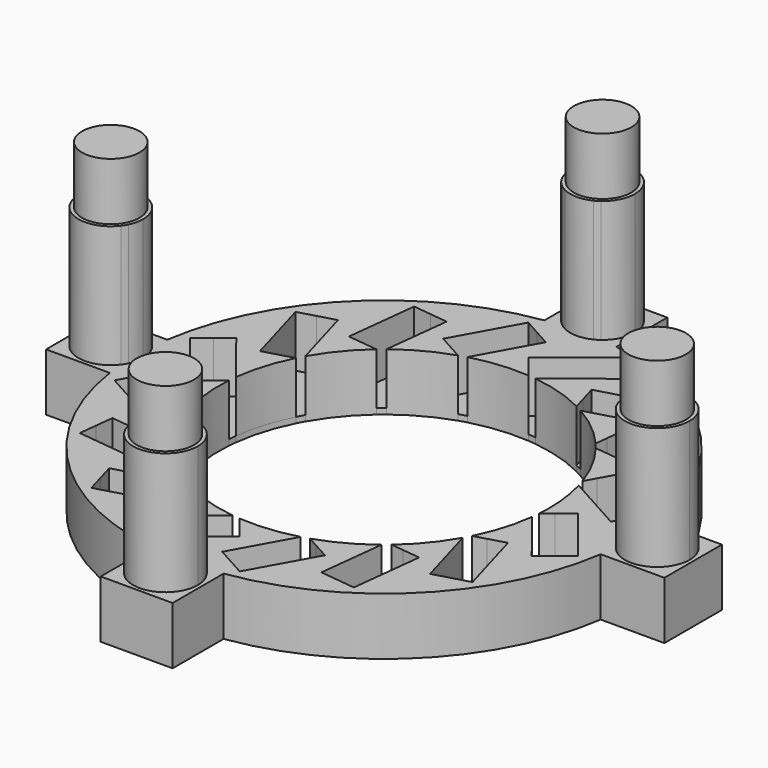
from build123d import *

# Parameters (mm, degrees)
F2_DEPTH = 8
F1_R     = 4
F3_DEPTH = 25
F4_DEPTH = 33
F5_DEPTH = 4
F0_R     = 34
F6_DEPTH = 0.8


# Not quite as in the source:
# - a feature names something its author has since deleted; it is built from what else it names


with BuildPart() as f2:
    # F1 (on Top) → F2 (new body)
    with BuildSketch(Plane.XY):
        with BuildLine():
            ThreePointArc((-33.944079, -1.949232), (-34.1514, -2.332012), (-34.394737, -2.692968))
            ThreePointArc((-34.394737, -2.692968), (-34.284658, -3.848663), (-34.135758, -5))
            ThreePointArc((-34.135758, -5), (-24.395184, -24.395184), (-5, -34.135758))
            ThreePointArc((-5, -34.135758), (-3.848663, -34.284658), (-2.692968, -34.394737))
            ThreePointArc((-2.692968, -34.394737), (-2.332012, -34.1514), (-1.949232, -33.944079))
            ThreePointArc((-1.949232, -33.944079), (-24.041631, -24.041631), (-33.944079, -1.949232))
        make_face()
        with BuildLine():
            ThreePointArc((-34.135758, -5), (-34.284658, -3.848663), (-34.394737, -2.692968))
            ThreePointArc((-34.394737, -2.692968), (-42.5, 0), (-34.394737, 2.692968))
            ThreePointArc((-34.394737, 2.692968), (-34.284658, 3.848663), (-34.135758, 5))
            Line((-34.135758, 5), (-43, 5))
            Line((-43, 5), (-43, 0))
            Line((-43, 0), (-43, -5))
            Line((-43, -5), (-34.135758, -5))
        make_face()
        with BuildLine():
            ThreePointArc((-34.135758, 5), (-34.284658, 3.848663), (-34.394737, 2.692968))
            ThreePointArc((-34.394737, 2.692968), (-34.1514, 2.332012), (-33.944079, 1.949232))
            ThreePointArc((-33.944079, 1.949232), (-24.041631, 24.041631), (-1.949232, 33.944079))
            ThreePointArc((-1.949232, 33.944079), (-2.332012, 34.1514), (-2.692968, 34.394737))
            ThreePointArc((-2.692968, 34.394737), (-3.848663, 34.284658), (-5, 34.135758))
            ThreePointArc((-5, 34.135758), (-24.395184, 24.395184), (-34.135758, 5))
        make_face()
        with BuildLine():
            ThreePointArc((-2.692968, -34.394737), (-3.848663, -34.284658), (-5, -34.135758))
            Line((-5, -34.135758), (-5, -43))
            Line((-5, -43), (0, -43))
            Line((0, -43), (5, -43))
            Line((5, -43), (5, -34.135758))
            ThreePointArc((5, -34.135758), (3.848663, -34.284658), (2.692968, -34.394737))
            ThreePointArc((2.692968, -34.394737), (4.022956, -35.983612), (4.5, -38))
            ThreePointArc((4.5, -38), (-2.016388, -42.022956), (-2.692968, -34.394737))
        make_face()
        with BuildLine():
            Line((-5, 43), (-5, 34.135758))
            ThreePointArc((-5, 34.135758), (-3.848663, 34.284658), (-2.692968, 34.394737))
            ThreePointArc((-2.692968, 34.394737), (-4.270462, 39.418858), (0, 42.5))
            Line((0, 42.5), (0, 43))
            Line((0, 43), (-5, 43))
        make_face()
        with BuildLine():
            ThreePointArc((33.944079, -1.949232), (24.041631, -24.041631), (1.949232, -33.944079))
            ThreePointArc((1.949232, -33.944079), (2.332012, -34.1514), (2.692968, -34.394737))
            ThreePointArc((2.692968, -34.394737), (3.848663, -34.284658), (5, -34.135758))
            ThreePointArc((5, -34.135758), (24.395184, -24.395184), (34.135758, -5))
            ThreePointArc((34.135758, -5), (34.284658, -3.848663), (34.394737, -2.692968))
            ThreePointArc((34.394737, -2.692968), (34.1514, -2.332012), (33.944079, -1.949232))
        make_face()
        with BuildLine():
            ThreePointArc((2.692968, 34.394737), (2.332012, 34.1514), (1.949232, 33.944079))
            ThreePointArc((1.949232, 33.944079), (24.041631, 24.041631), (33.944079, 1.949232))
            ThreePointArc((33.944079, 1.949232), (34.1514, 2.332012), (34.394737, 2.692968))
            ThreePointArc((34.394737, 2.692968), (34.284658, 3.848663), (34.135758, 5))
            ThreePointArc((34.135758, 5), (24.395184, 24.395184), (5, 34.135758))
            ThreePointArc((5, 34.135758), (3.848663, 34.284658), (2.692968, 34.394737))
        make_face()
        with BuildLine():
            Line((0, 43), (0, 42.5))
            ThreePointArc((0, 42.5), (3.181981, 41.181981), (4.5, 38))
            ThreePointArc((4.5, 38), (4.022956, 35.983612), (2.692968, 34.394737))
            ThreePointArc((2.692968, 34.394737), (3.848663, 34.284658), (5, 34.135758))
            Line((5, 34.135758), (5, 43))
            Line((5, 43), (0, 43))
        make_face()
        with BuildLine():
            ThreePointArc((42.5, 0), (39.418858, -4.270462), (34.394737, -2.692968))
            ThreePointArc((34.394737, -2.692968), (34.284658, -3.848663), (34.135758, -5))
            Line((34.135758, -5), (43, -5))
            Line((43, -5), (43, 0))
            Line((43, 0), (43, 5))
            Line((43, 5), (34.135758, 5))
            ThreePointArc((34.135758, 5), (34.284658, 3.848663), (34.394737, 2.692968))
            ThreePointArc((34.394737, 2.692968), (39.418858, 4.270462), (42.5, 0))
        make_face()
        with BuildLine():
            ThreePointArc((-33.5, 0), (-33.612424, -0.999589), (-33.944079, -1.949232))
            ThreePointArc((-33.944079, -1.949232), (-24.041631, -24.041631), (-1.949232, -33.944079))
            ThreePointArc((-1.949232, -33.944079), (0, -33.5), (1.949232, -33.944079))
            ThreePointArc((1.949232, -33.944079), (24.041631, -24.041631), (33.944079, -1.949232))
            ThreePointArc((33.944079, -1.949232), (33.5, 0), (33.944079, 1.949232))
            ThreePointArc((33.944079, 1.949232), (24.041631, 24.041631), (1.949232, 33.944079))
            ThreePointArc((1.949232, 33.944079), (0, 33.5), (-1.949232, 33.944079))
            ThreePointArc((-1.949232, 33.944079), (-24.041631, 24.041631), (-33.944079, 1.949232))
            ThreePointArc((-33.944079, 1.949232), (-33.612424, 0.999589), (-33.5, 0))
        make_face()
        with BuildLine():
            ThreePointArc((22.165631, 6.138794), (22.790453, 3.097618), (23, 0))
            ThreePointArc((23, 0), (22.98399, -0.858012), (22.935984, -1.71483))
            Line((22.935984, -1.71483), (24.292118, -0.636112))
            Line((24.292118, -0.636112), (26.248639, 0.920175))
            Line((26.248639, 0.920175), (32.473785, -6.905906))
            Line((32.473785, -6.905906), (30.517265, -8.462193))
            Line((30.517265, -8.462193), (28.560744, -10.01848))
            Line((28.560744, -10.01848), (22.827588, -2.810914))
            ThreePointArc((22.827588, -2.810914), (22.006964, -6.685323), (20.533849, -10.361517))
            Line((20.533849, -10.361517), (22.199562, -9.883882))
            Line((22.199562, -9.883882), (24.602716, -9.194788))
            Line((24.602716, -9.194788), (27.35909, -18.807405))
            Line((27.35909, -18.807405), (24.955935, -19.496499))
            Line((24.955935, -19.496499), (22.552781, -20.185592))
            Line((22.552781, -20.185592), (20.014251, -11.332685))
            ThreePointArc((20.014251, -11.332685), (17.773421, -14.598134), (15.005622, -17.430757))
            Line((15.005622, -17.430757), (16.727323, -17.62692))
            Line((16.727323, -17.62692), (19.211253, -17.909928))
            Line((19.211253, -17.909928), (18.07922, -27.845647))
            Line((18.07922, -27.845647), (15.595291, -27.562639))
            Line((15.595291, -27.562639), (13.111361, -27.279631))
            Line((13.111361, -27.279631), (14.153926, -18.129158))
            ThreePointArc((14.153926, -18.129158), (10.834036, -20.288511), (7.192925, -21.846323))
            Line((7.192925, -21.846323), (8.708501, -22.68642))
            Line((8.708501, -22.68642), (10.89505, -23.898444))
            Line((10.89505, -23.898444), (6.046954, -32.644642))
            Line((6.046954, -32.644642), (3.860405, -31.432617))
            Line((3.860405, -31.432617), (1.673855, -30.220593))
            Line((1.673855, -30.220593), (6.138794, -22.165631))
            ThreePointArc((6.138794, -22.165631), (2.245267, -22.890146), (-1.71483, -22.935984))
            Line((-1.71483, -22.935984), (-0.636112, -24.292118))
            Line((-0.636112, -24.292118), (0.920175, -26.248639))
            Line((0.920175, -26.248639), (-6.905906, -32.473785))
            Line((-6.905906, -32.473785), (-8.462193, -30.517265))
            Line((-8.462193, -30.517265), (-10.01848, -28.560744))
            Line((-10.01848, -28.560744), (-2.810914, -22.827588))
            ThreePointArc((-2.810914, -22.827588), (-6.685323, -22.006964), (-10.361517, -20.533849))
            Line((-10.361517, -20.533849), (-9.883882, -22.199562))
            Line((-9.883882, -22.199562), (-9.194788, -24.602716))
            Line((-9.194788, -24.602716), (-18.807405, -27.35909))
            Line((-18.807405, -27.35909), (-19.496499, -24.955935))
            Line((-19.496499, -24.955935), (-20.185592, -22.552781))
            Line((-20.185592, -22.552781), (-11.332685, -20.014251))
            ThreePointArc((-11.332685, -20.014251), (-14.598134, -17.773421), (-17.430757, -15.005622))
            Line((-17.430757, -15.005622), (-17.62692, -16.727323))
            Line((-17.62692, -16.727323), (-17.909928, -19.211253))
            Line((-17.909928, -19.211253), (-27.845647, -18.07922))
            Line((-27.845647, -18.07922), (-27.562639, -15.595291))
            Line((-27.562639, -15.595291), (-27.279631, -13.111361))
            Line((-27.279631, -13.111361), (-18.129158, -14.153926))
            ThreePointArc((-18.129158, -14.153926), (-20.288511, -10.834036), (-21.846323, -7.192925))
            Line((-21.846323, -7.192925), (-22.68642, -8.708501))
            Line((-22.68642, -8.708501), (-23.898444, -10.89505))
            Line((-23.898444, -10.89505), (-32.644642, -6.046954))
            Line((-32.644642, -6.046954), (-31.432617, -3.860405))
            Line((-31.432617, -3.860405), (-30.220593, -1.673855))
            Line((-30.220593, -1.673855), (-22.165631, -6.138794))
            ThreePointArc((-22.165631, -6.138794), (-22.890146, -2.245267), (-22.935984, 1.71483))
            Line((-22.935984, 1.71483), (-24.292118, 0.636112))
            Line((-24.292118, 0.636112), (-26.248639, -0.920175))
            Line((-26.248639, -0.920175), (-32.473785, 6.905906))
            Line((-32.473785, 6.905906), (-30.517265, 8.462193))
            Line((-30.517265, 8.462193), (-28.560744, 10.01848))
            Line((-28.560744, 10.01848), (-22.827588, 2.810914))
            ThreePointArc((-22.827588, 2.810914), (-22.006964, 6.685323), (-20.533849, 10.361517))
            Line((-20.533849, 10.361517), (-22.199562, 9.883882))
            Line((-22.199562, 9.883882), (-24.602716, 9.194788))
            Line((-24.602716, 9.194788), (-27.35909, 18.807405))
            Line((-27.35909, 18.807405), (-24.955935, 19.496499))
            Line((-24.955935, 19.496499), (-22.552781, 20.185592))
            Line((-22.552781, 20.185592), (-20.014251, 11.332685))
            ThreePointArc((-20.014251, 11.332685), (-17.773421, 14.598134), (-15.005622, 17.430757))
            Line((-15.005622, 17.430757), (-16.727323, 17.62692))
            Line((-16.727323, 17.62692), (-19.211253, 17.909928))
            Line((-19.211253, 17.909928), (-18.07922, 27.845647))
            Line((-18.07922, 27.845647), (-15.595291, 27.562639))
            Line((-15.595291, 27.562639), (-13.111361, 27.279631))
            Line((-13.111361, 27.279631), (-14.153926, 18.129158))
            ThreePointArc((-14.153926, 18.129158), (-10.834036, 20.288511), (-7.192925, 21.846323))
            Line((-7.192925, 21.846323), (-8.708501, 22.68642))
            Line((-8.708501, 22.68642), (-10.89505, 23.898444))
            Line((-10.89505, 23.898444), (-6.046954, 32.644642))
            Line((-6.046954, 32.644642), (-3.860405, 31.432617))
            Line((-3.860405, 31.432617), (-1.673855, 30.220593))
            Line((-1.673855, 30.220593), (-6.138794, 22.165631))
            ThreePointArc((-6.138794, 22.165631), (-2.245267, 22.890146), (1.71483, 22.935984))
            Line((1.71483, 22.935984), (0.636112, 24.292118))
            Line((0.636112, 24.292118), (-0.920175, 26.248639))
            Line((-0.920175, 26.248639), (6.905906, 32.473785))
            Line((6.905906, 32.473785), (8.462193, 30.517265))
            Line((8.462193, 30.517265), (10.01848, 28.560744))
            Line((10.01848, 28.560744), (2.810914, 22.827588))
            ThreePointArc((2.810914, 22.827588), (6.685323, 22.006964), (10.361517, 20.533849))
            Line((10.361517, 20.533849), (9.883882, 22.199562))
            Line((9.883882, 22.199562), (9.194788, 24.602716))
            Line((9.194788, 24.602716), (18.807405, 27.35909))
            Line((18.807405, 27.35909), (19.496499, 24.955935))
            Line((19.496499, 24.955935), (20.185592, 22.552781))
            Line((20.185592, 22.552781), (11.332685, 20.014251))
            ThreePointArc((11.332685, 20.014251), (14.598134, 17.773421), (17.430757, 15.005622))
            Line((17.430757, 15.005622), (17.62692, 16.727323))
            Line((17.62692, 16.727323), (17.909928, 19.211253))
            Line((17.909928, 19.211253), (27.845647, 18.07922))
            Line((27.845647, 18.07922), (27.562639, 15.595291))
            Line((27.562639, 15.595291), (27.279631, 13.111361))
            Line((27.279631, 13.111361), (18.129158, 14.153926))
            ThreePointArc((18.129158, 14.153926), (20.288511, 10.834036), (21.846323, 7.192925))
            Line((21.846323, 7.192925), (22.68642, 8.708501))
            Line((22.68642, 8.708501), (23.898444, 10.89505))
            Line((23.898444, 10.89505), (32.644642, 6.046954))
            Line((32.644642, 6.046954), (31.432617, 3.860405))
            Line((31.432617, 3.860405), (30.220593, 1.673855))
            Line((30.220593, 1.673855), (22.165631, 6.138794))
        make_face(mode=Mode.SUBTRACT)
    extrude(amount=F2_DEPTH)

    # F1 (on Top) → F3 (join)
    with BuildSketch(Plane.XY):
        with BuildLine():
            ThreePointArc((-2.692968, 34.394737), (-2.332012, 34.1514), (-1.949232, 33.944079))
            ThreePointArc((-1.949232, 33.944079), (0, 33.5), (1.949232, 33.944079))
            ThreePointArc((1.949232, 33.944079), (2.332012, 34.1514), (2.692968, 34.394737))
            ThreePointArc((2.692968, 34.394737), (4.022956, 35.983612), (4.5, 38))
            ThreePointArc((4.5, 38), (3.181981, 41.181981), (0, 42.5))
            ThreePointArc((0, 42.5), (-4.270462, 39.418858), (-2.692968, 34.394737))
        make_face()
        with Locations((0, 38)):
            Circle(F1_R, mode=Mode.SUBTRACT)
        with BuildLine():
            ThreePointArc((33.944079, 1.949232), (33.5, 0), (33.944079, -1.949232))
            ThreePointArc((33.944079, -1.949232), (34.1514, -2.332012), (34.394737, -2.692968))
            ThreePointArc((34.394737, -2.692968), (39.418858, -4.270462), (42.5, 0))
            ThreePointArc((42.5, 0), (39.418858, 4.270462), (34.394737, 2.692968))
            ThreePointArc((34.394737, 2.692968), (34.1514, 2.332012), (33.944079, 1.949232))
        make_face()
        with Locations((38, 0)):
            Circle(F1_R, mode=Mode.SUBTRACT)
        with BuildLine():
            ThreePointArc((1.949232, -33.944079), (0, -33.5), (-1.949232, -33.944079))
            ThreePointArc((-1.949232, -33.944079), (-2.332012, -34.1514), (-2.692968, -34.394737))
            ThreePointArc((-2.692968, -34.394737), (-2.016388, -42.022956), (4.5, -38))
            ThreePointArc((4.5, -38), (4.022956, -35.983612), (2.692968, -34.394737))
            ThreePointArc((2.692968, -34.394737), (2.332012, -34.1514), (1.949232, -33.944079))
        make_face()
        with Locations((0, -38)):
            Circle(F1_R, mode=Mode.SUBTRACT)
        with BuildLine():
            ThreePointArc((-34.394737, 2.692968), (-42.5, 0), (-34.394737, -2.692968))
            ThreePointArc((-34.394737, -2.692968), (-34.1514, -2.332012), (-33.944079, -1.949232))
            ThreePointArc((-33.944079, -1.949232), (-33.612424, -0.999589), (-33.5, 0))
            ThreePointArc((-33.5, 0), (-33.612424, 0.999589), (-33.944079, 1.949232))
            ThreePointArc((-33.944079, 1.949232), (-34.1514, 2.332012), (-34.394737, 2.692968))
        make_face()
        with Locations((-38, 0)):
            Circle(F1_R, mode=Mode.SUBTRACT)
        with Locations((0, 38)):
            Circle(F1_R)
        with Locations((38, 0)):
            Circle(F1_R)
        with Locations((0, -38)):
            Circle(F1_R)
        with Locations((-38, 0)):
            Circle(F1_R)
    extrude(amount=F3_DEPTH)

    # F1 (on Top) → F4 (join)
    with BuildSketch(Plane.XY):
        with Locations((38, 0)):
            Circle(F1_R)
        with Locations((0, -38)):
            Circle(F1_R)
        with Locations((0, 38)):
            Circle(F1_R)
        with Locations((-38, 0)):
            Circle(F1_R)
    extrude(amount=F4_DEPTH)

    # F1 (on Top) → F5 (cut)
    with BuildSketch(Plane.XY):
        with Locations((-38, 0)):
            Circle(F1_R)
        with Locations((38, 0)):
            Circle(F1_R)
        with Locations((0, 38)):
            Circle(F1_R)
        with Locations((0, -38)):
            Circle(F1_R)
    extrude(amount=F5_DEPTH, mode=Mode.SUBTRACT)

    # F0 (on Top) → F6 (join)
    with BuildSketch(Plane.XY):
        Circle(F0_R)
        with BuildLine():
            ThreePointArc((2.810914, 22.827588), (17.228625, 15.237273), (23, 0))
            ThreePointArc((23, 0), (-16.858842, -15.645429), (1.71483, 22.935984))
            Line((1.71483, 22.935984), (0.636112, 24.292118))
            Line((0.636112, 24.292118), (-0.920175, 26.248639))
            Line((-0.920175, 26.248639), (6.905906, 32.473785))
            Line((6.905906, 32.473785), (8.462193, 30.517265))
            Line((8.462193, 30.517265), (10.01848, 28.560744))
            Line((10.01848, 28.560744), (2.810914, 22.827588))
        make_face(mode=Mode.SUBTRACT)
        with BuildLine():
            ThreePointArc((1.71483, 22.935984), (2.263521, 22.888348), (2.810914, 22.827588))
            Line((2.810914, 22.827588), (10.01848, 28.560744))
            Line((10.01848, 28.560744), (8.462193, 30.517265))
            Line((8.462193, 30.517265), (6.905906, 32.473785))
            Line((6.905906, 32.473785), (-0.920175, 26.248639))
            Line((-0.920175, 26.248639), (0.636112, 24.292118))
            Line((0.636112, 24.292118), (1.71483, 22.935984))
        make_face()
    extrude(amount=F6_DEPTH)


solid = f2.part
